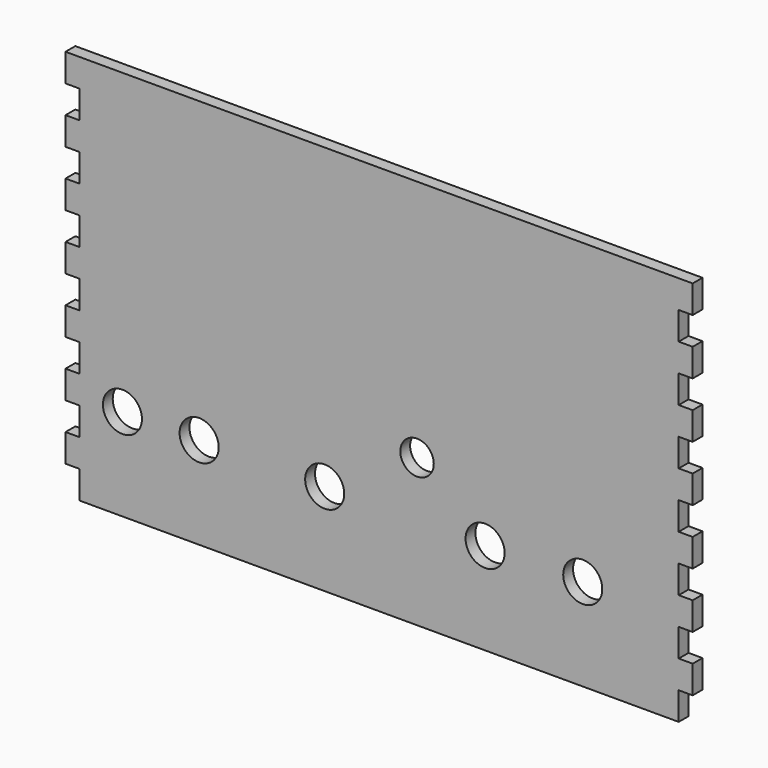
from build123d import *

# Parameters (mm, degrees)
F0_W     = 285.496
F0_H     = 177.8
F1_DEPTH = 5.588
F3_D     = 17.78
F4_W     = 6.35
F4_H     = 12.7
F5_DEPTH = 25.4
F6_R     = 7.62
F7_DEPTH = 25.4


# Not quite as in the source:
# - a pattern or mirror of a feature is missing from the dataset's text; its kind, count and spacing are read off the source's solid


with BuildPart() as f1:
    # F0 (on Front) → F1 (new body)
    with BuildSketch(Plane.XZ):
        Rectangle(F0_W, F0_H)
    extrude(amount=F1_DEPTH)

    # F3 (through all)
    with Locations(Plane(origin=(0, 0, 0), x_dir=(1, 0, 0), z_dir=(0, 1, 0))):
        with Locations((-116.84, 46.99), (-81.915, 46.99), (-24.765, 46.99), (48.26, 46.99), (92.71, 46.99)):
            Hole(F3_D / 2)

    # F4 (on Front) → F5 (cut)
    with BuildSketch(Plane.XZ):
        with Locations((139.573, 69.85)):
            Rectangle(F4_W, F4_H)
        with Locations((139.573, 44.45)):
            Rectangle(F4_W, F4_H)
        with Locations((139.573, 19.05)):
            Rectangle(F4_W, F4_H)
        with Locations((139.573, -6.35)):
            Rectangle(F4_W, F4_H)
        with Locations((139.573, -31.75)):
            Rectangle(F4_W, F4_H)
        with Locations((139.573, -57.15)):
            Rectangle(F4_W, F4_H)
        with Locations((139.573, -82.55)):
            Rectangle(F4_W, F4_H)
    f5 = extrude(amount=F5_DEPTH, mode=Mode.SUBTRACT)

    # F5_copies: F5 across plane
    add(f5.mirror(Plane(origin=(0, 0, 0), x_dir=(0, 0, -1), z_dir=(-1, 0, 0))), mode=Mode.SUBTRACT)

    # F6 (on Front) → F7 (cut)
    with BuildSketch(Plane.XZ):
        with Locations((17.272, -21.7023361474)):
            Circle(F6_R)
    extrude(amount=F7_DEPTH, mode=Mode.SUBTRACT)


solid = f1.part
